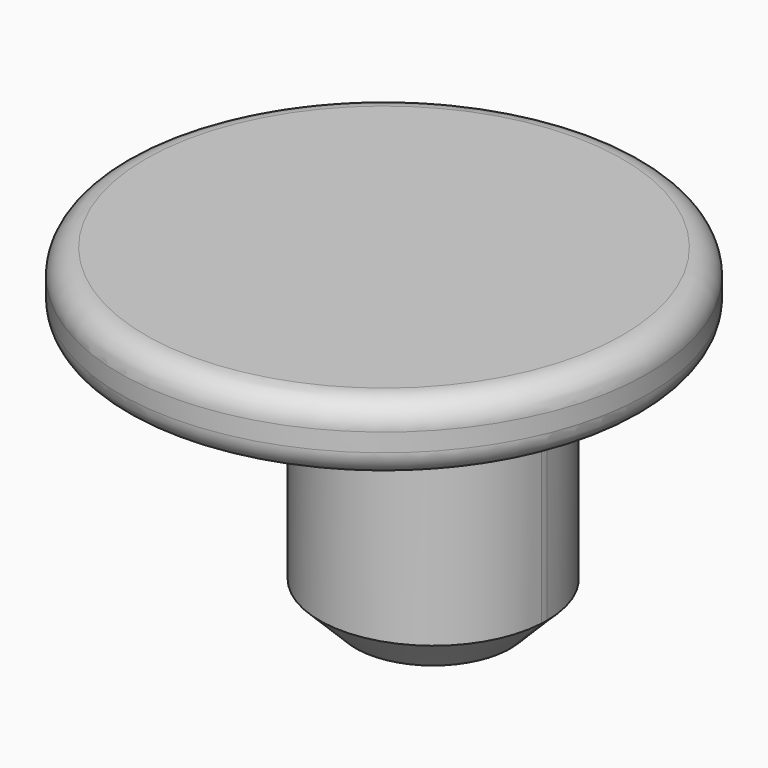
from build123d import *

# Parameters (mm, degrees)
F1_DEPTH = 7.8
F0_R     = 7.25
F2_DEPTH = 1.9
F3_SIZE  = 1
F4_R     = 0.7


# Not quite as in the source:
# - a feature names something its author has since deleted; it is built from what else it names


with BuildPart() as f1:
    # F0 (on Top) → F1 (new body)
    with BuildSketch(Plane.XY):
        with BuildLine():
            ThreePointArc((1.8904761229, -0.1900000758), (0, -1.9), (-1.8904761229, -0.1900000758))
            Line((-1.8904761229, -0.1900000758), (-3.1192186475, -0.1900000758))
            ThreePointArc((-3.1192186475, -0.1900000758), (0, -3.125), (3.1192186475, -0.1900000758))
            Line((3.1192186475, -0.1900000758), (1.8904761229, -0.1900000758))
        make_face()
        with BuildLine():
            ThreePointArc((-1.8904761229, -0.1900000758), (-0.0951193107, 1.897617537), (1.9, 0))
            ThreePointArc((1.9, 0), (1.897617537, -0.0951193107), (1.8904761229, -0.1900000758))
            Line((1.8904761229, -0.1900000758), (3.1192186475, -0.1900000758))
            ThreePointArc((3.1192186475, -0.1900000758), (3.1235543275, -0.0950440067), (3.125, 0))
            ThreePointArc((3.125, 0), (-0.0950440067, 3.1235543275), (-3.1192186475, -0.1900000758))
            Line((-3.1192186475, -0.1900000758), (-1.8904761229, -0.1900000758))
        make_face()
    extrude(amount=-F1_DEPTH)

    # F0 (on Top) → F2 (join)
    with BuildSketch(Plane.XY):
        with Locations((2.98e-08, -1.6900000758)):
            Circle(F0_R)
        Polygon((2.5797043927, -5.2021308802), (0, -7.9360147938), (-2.5797043927, -5.2021308802), align=None, mode=Mode.SUBTRACT)
        with BuildLine():
            Line((-5.4999999702, -0.1900000758), (-3.1192186475, -0.1900000758))
            ThreePointArc((-3.1192186475, -0.1900000758), (-0.0950440067, 3.1235543275), (3.125, 0))
            ThreePointArc((3.125, 0), (3.1235543275, -0.0950440067), (3.1192186475, -0.1900000758))
            Line((3.1192186475, -0.1900000758), (5.5000000298, -0.1900000758))
            Line((5.5000000298, -0.1900000758), (5.5000000298, -3.1900000758))
            Line((5.5000000298, -3.1900000758), (-5.4999999702, -3.1900000758))
            Line((-5.4999999702, -3.1900000758), (-5.4999999702, -0.1900000758))
        make_face(mode=Mode.SUBTRACT)
        with BuildLine():
            ThreePointArc((3.1192186475, -0.1900000758), (0, -3.125), (-3.1192186475, -0.1900000758))
            Line((-3.1192186475, -0.1900000758), (-5.4999999702, -0.1900000758))
            Line((-5.4999999702, -0.1900000758), (-5.4999999702, -3.1900000758))
            Line((-5.4999999702, -3.1900000758), (5.5000000298, -3.1900000758))
            Line((5.5000000298, -3.1900000758), (5.5000000298, -0.1900000758))
            Line((5.5000000298, -0.1900000758), (3.1192186475, -0.1900000758))
        make_face()
        with BuildLine():
            ThreePointArc((-1.8904761229, -0.1900000758), (-0.0951193107, 1.897617537), (1.9, 0))
            ThreePointArc((1.9, 0), (1.897617537, -0.0951193107), (1.8904761229, -0.1900000758))
            Line((1.8904761229, -0.1900000758), (3.1192186475, -0.1900000758))
            ThreePointArc((3.1192186475, -0.1900000758), (3.1235543275, -0.0950440067), (3.125, 0))
            ThreePointArc((3.125, 0), (-0.0950440067, 3.1235543275), (-3.1192186475, -0.1900000758))
            Line((-3.1192186475, -0.1900000758), (-1.8904761229, -0.1900000758))
        make_face()
        with BuildLine():
            ThreePointArc((1.8904761229, -0.1900000758), (0, -1.9), (-1.8904761229, -0.1900000758))
            Line((-1.8904761229, -0.1900000758), (-3.1192186475, -0.1900000758))
            ThreePointArc((-3.1192186475, -0.1900000758), (0, -3.125), (3.1192186475, -0.1900000758))
            Line((3.1192186475, -0.1900000758), (1.8904761229, -0.1900000758))
        make_face()
        Polygon((-2.5797043927, -5.2021308802), (0, -7.9360147938), (2.5797043927, -5.2021308802), align=None)
        with BuildLine():
            ThreePointArc((1.8904761229, -0.1900000758), (1.897617537, -0.0951193107), (1.9, 0))
            ThreePointArc((1.9, 0), (-0.0951193107, 1.897617537), (-1.8904761229, -0.1900000758))
            Line((-1.8904761229, -0.1900000758), (1.8904761229, -0.1900000758))
        make_face()
        with BuildLine():
            Line((1.8904761229, -0.1900000758), (-1.8904761229, -0.1900000758))
            ThreePointArc((-1.8904761229, -0.1900000758), (0, -1.9), (1.8904761229, -0.1900000758))
        make_face()
    extrude(amount=F2_DEPTH)

    # F3
    f3_edges = [f1.edges().sort_by_distance(p)[0] for p in [
        (3.119219, 0.19, -7.8),
    ]]
    chamfer(f3_edges, length=F3_SIZE)

    # F4
    f4_edges = [f1.edges().sort_by_distance(p)[0] for p in [
        (-7.25, -1.69, 0),
        (-7.25, -1.69, 1.9),
    ]]
    fillet(f4_edges, radius=F4_R)


solid = f1.part
